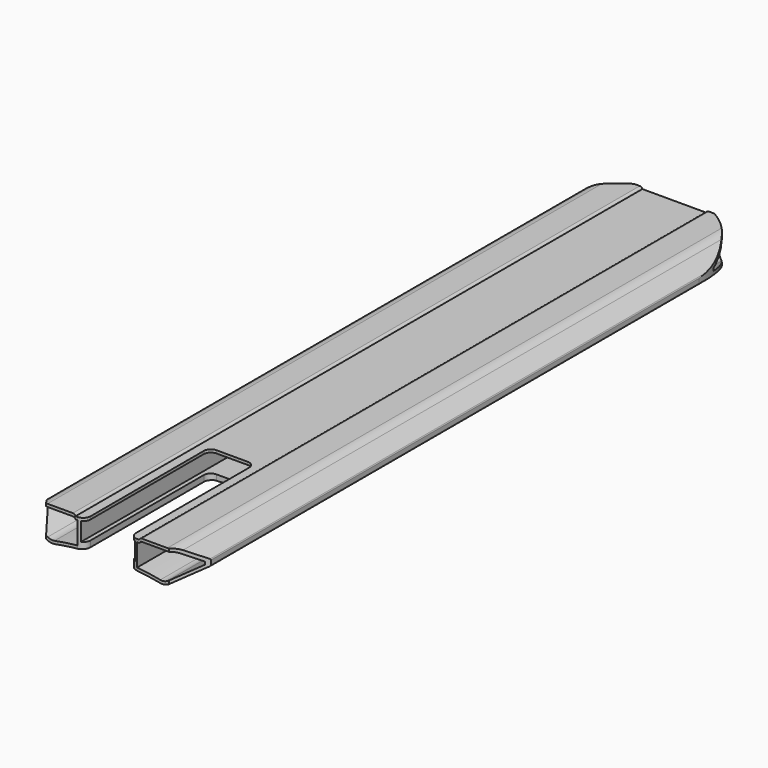
from build123d import *

# Parameters (mm, degrees)
F2_DEPTH       = 250
F3_W           = 38
F3_H           = 13
F4_DEPTH       = 250
F5_R           = 9
F6_R           = 1
F7_T1_DEPTH    = 509.3674969976
F9_DEPTH       = 500.001
F12_DEPTH      = 13.5192964571
F12_DEPTH_BACK = 10.001
F13_T1_DEPTH   = 2
F13_T6_DEPTH   = 16.7634354909
F13_S7_R       = 200
F13_T8_DEPTH   = 11
F13_T12_DEPTH  = 16.7632527384
F13_S13_R      = 200
F13_T14_DEPTH  = 11
F13_T15_DEPTH  = 29.2634354909
F13_T17_DEPTH  = 27
F13_T19_DEPTH  = 29.2632527384
F14_DEPTH      = 13.5192964571
F14_DEPTH_BACK = 10.001


# Not quite as in the source:
# - a fillet or chamfer that OpenCascade refuses, or shapes differently, is made with other operations: its cross-section is extruded or revolved along the edge and cut away or added


with BuildPart() as f2:
    # F0 (on Front) → F2 (new body, symmetric)
    with BuildSketch(Plane.XZ):
        with BuildLine():
            Line((-22.5004640741, 10), (-45.5824640741, 10))
            Line((-45.5824640741, 10), (-57.5, 0))
            Line((-57.5, 0), (-57.5, -4))
            Line((-57.5, -4), (-40.1794919243, -14))
            ThreePointArc((-40.1794919243, -14), (0.0006744682, -9.9223168214), (40.1808408606, -14))
            Line((40.1808408606, -14), (57.5, -4.0007788087))
            Line((57.5, -4.0007788087), (57.5, -0.0007788087))
            Line((57.5, -0.0007788087), (45.5815359259, 10))
            Line((45.5815359259, 10), (22.4995359259, 10))
            Line((22.4995359259, 10), (22.4995359259, 8.7))
            Line((22.4995359259, 8.7), (-22.5004640741, 8.7))
            Line((-22.5004640741, 8.7), (-22.5004640741, 10))
        make_face()
    extrude(amount=F2_DEPTH, both=True)

    # F3 (on Front) → F4 (cut, symmetric)
    with BuildSketch(Plane.XZ):
        with Locations((0, 0.2)):
            Rectangle(F3_W, F3_H)
    extrude(amount=F4_DEPTH, both=True, mode=Mode.SUBTRACT)

    # F5
    f5_edges = [f2.edges().sort_by_distance(p)[0] for p in [
        (45.581536, 0, 10),
        (40.180841, 0, -14),
        (-45.582464, 0, 10),
        (-40.179492, 0, -14),
    ]]
    fillet(f5_edges, radius=F5_R)

    # F6
    f6_edges = [f2.edges().sort_by_distance(p)[0] for p in [
        (57.5, 0, -0.000779),
        (57.5, 0, -4.000779),
        (-57.5, 0, 0),
        (-57.5, 0, -4),
    ]]
    fillet(f6_edges, radius=F6_R)

    # F7: fillet of radius 2 on 2 edges, made by hand

    # F7_s2 → F7_t1 (cut)
    with BuildSketch(Plane.XZ.offset(-254.6837484988)):
        with BuildLine():
            ThreePointArc((24.3730353255, 10), (23.2328599004, 9.6431676725), (22.4995359259, 8.7))
            Line((22.4995359259, 8.7), (22.4995359259, 10))
            Line((22.4995359259, 10), (24.3730353255, 10))
        make_face()
        with BuildLine():
            ThreePointArc((-22.5004640741, 8.7), (-23.2337880485, 9.6431676725), (-24.3739634736, 10))
            Line((-24.3739634736, 10), (-22.5004640741, 10))
            Line((-22.5004640741, 10), (-22.5004640741, 8.7))
        make_face()
    extrude(amount=F7_T1_DEPTH, mode=Mode.SUBTRACT)

    # F8 (on face) → F9 (cut, through all)
    with BuildSketch(Plane.XZ.offset(250)):
        with BuildLine():
            Line((-21, -9.0169369236), (-21, 6.6999997944))
            Line((-21, 6.6999997944), (-22.5004640741, 6.6999997944))
            ThreePointArc((-22.5004640741, 6.6999997944), (-23.2337879899, 7.6431676078), (-24.3739634736, 8))
            Line((-24.3739634736, 8), (-42.3067319657, 8))
            ThreePointArc((-42.3067319657, 8), (-44.7008729689, 7.5778483455), (-46.8062452335, 6.3623111018))
            Line((-46.8062452335, 6.3623111018), (-55.5, -0.9326153163))
            Line((-55.5, -0.9326153163), (-55.5, -2.8452994616))
            Line((-55.5, -2.8452994616), (-42.102284203, -10.5804742836))
            ThreePointArc((-42.102284203, -10.5804742836), (-39.7790708711, -11.4186713119), (-37.3093621422, -11.3978569477))
            ThreePointArc((-37.3093621422, -11.3978569477), (-29.178975147, -10.0409819041), (-21, -9.0169369236))
        make_face()
        with BuildLine():
            Line((22.5004640741, 6.6999997944), (21, 6.6999997944))
            Line((21, 6.6999997944), (21, -9.0169369236))
            ThreePointArc((21, -9.0169369236), (29.178975147, -10.0409819041), (37.3093621422, -11.3978569477))
            ThreePointArc((37.3093621422, -11.3978569477), (39.7790708711, -11.4186713119), (42.102284203, -10.5804742836))
            Line((42.102284203, -10.5804742836), (55.5, -2.8452994616))
            Line((55.5, -2.8452994616), (55.5, -0.9326153163))
            Line((55.5, -0.9326153163), (46.8062452335, 6.3623111018))
            ThreePointArc((46.8062452335, 6.3623111018), (44.7008729689, 7.5778483455), (42.3067319657, 8))
            Line((42.3067319657, 8), (24.3739634736, 8))
            ThreePointArc((24.3739634736, 8), (23.2337879899, 7.6431676078), (22.5004640741, 6.6999997944))
        make_face()
    extrude(amount=-F9_DEPTH, mode=Mode.SUBTRACT)

    # F11 (on Top) → F12 (cut, two sides)
    with BuildSketch(Plane.XY) as f12_sk:
        Polygon((-68.0004640741, -346), (67.9995359259, -346), (67.9995359259, -216), (43.2970899738, -250), (15.9995359259, -250), (15.9995359259, -140), (-16.0004640741, -140), (-16.0004640741, -250), (-43.2980181219, -250), (-68.0004640741, -216), align=None)
    extrude(amount=-F12_DEPTH, mode=Mode.SUBTRACT)
    extrude(f12_sk.sketch, amount=F12_DEPTH_BACK, mode=Mode.SUBTRACT)

    # F13: fillet of radius 5 on 8 edges, made by hand

    # F13_s2 → F13_t1 (join)
    with BuildSketch(Plane.XY.offset(6.7)):
        with BuildLine():
            ThreePointArc((-11.0004640741, -140), (-14.53599798, -141.4644660941), (-16.0004640741, -145))
            Line((-16.0004640741, -145), (-16.0004640741, -140))
            Line((-16.0004640741, -140), (-11.0004640741, -140))
        make_face()
        with BuildLine():
            ThreePointArc((15.9995359259, -145), (14.5350698319, -141.4644660941), (10.9995359259, -140))
            Line((10.9995359259, -140), (15.9995359259, -140))
            Line((15.9995359259, -140), (15.9995359259, -145))
        make_face()
    extrude(amount=F13_T1_DEPTH)


with BuildPart() as f13_tool4:
    # F13_s5 → F13_t6 (new body)
    with BuildSketch(Plane.XY.offset(-23.0634354909)):
        with BuildLine():
            ThreePointArc((-16.0004640741, -145), (-14.53599798, -141.4644660941), (-11.0004640741, -140))
            Line((-11.0004640741, -140), (-16.0004640741, -140))
            Line((-16.0004640741, -140), (-16.0004640741, -145))
        make_face()
    extrude(amount=F13_T6_DEPTH)

    # F13_s7 → F13_t8 (cut, symmetric)
    with BuildSketch(Plane.XZ.offset(142.5)):
        with Locations((0.0006744682, -209.9223168214)):
            Circle(F13_S7_R)
    extrude(amount=F13_T8_DEPTH, both=True, mode=Mode.SUBTRACT)


with BuildPart() as f2_1:
    add(f2.part)

    # F13_t3: union F13_tool4
    add(f13_tool4.part)


with BuildPart() as f13_tool10:
    # F13_s11 → F13_t12 (new body)
    with BuildSketch(Plane.XY.offset(-23.0632527384)):
        with BuildLine():
            ThreePointArc((15.9995359259, -145), (14.5350698319, -141.4644660941), (10.9995359259, -140))
            Line((10.9995359259, -140), (15.9995359259, -140))
            Line((15.9995359259, -140), (15.9995359259, -145))
        make_face()
    extrude(amount=F13_T12_DEPTH)

    # F13_s13 → F13_t14 (cut, symmetric)
    with BuildSketch(Plane.XZ.offset(142.5)):
        with Locations((0.0006744682, -209.9223168214)):
            Circle(F13_S13_R)
    extrude(amount=F13_T14_DEPTH, both=True, mode=Mode.SUBTRACT)


with BuildPart() as f2_2:
    add(f2_1.part)

    # F13_t9: union F13_tool10
    add(f13_tool10.part)

    # F13_s16 → F13_t15 (cut)
    with BuildSketch(Plane.XY.offset(-23.0634354909)):
        with BuildLine():
            ThreePointArc((-21.0004640741, -250), (-17.4649301681, -248.5355339059), (-16.0004640741, -245))
            Line((-16.0004640741, -245), (-16.0004640741, -250))
            Line((-16.0004640741, -250), (-21.0004640741, -250))
        make_face()
    extrude(amount=F13_T15_DEPTH, mode=Mode.SUBTRACT)

    # F13_s18 → F13_t17 (cut)
    with BuildSketch(Plane.XY.offset(-5.8)):
        with BuildLine():
            ThreePointArc((20.9995359259, -250), (17.46400202, -248.5355339059), (15.9995359259, -245))
            Line((15.9995359259, -245), (15.9995359259, -250))
            Line((15.9995359259, -250), (20.9995359259, -250))
        make_face()
        with BuildLine():
            ThreePointArc((-16.0004640741, -245), (-17.4649301681, -248.5355339059), (-21.0004640741, -250))
            Line((-21.0004640741, -250), (-16.0004640741, -250))
            Line((-16.0004640741, -250), (-16.0004640741, -245))
        make_face()
    extrude(amount=F13_T17_DEPTH, mode=Mode.SUBTRACT)

    # F13_s20 → F13_t19 (cut)
    with BuildSketch(Plane.XY.offset(-23.0632527384)):
        with BuildLine():
            ThreePointArc((20.9995359259, -250), (17.46400202, -248.5355339059), (15.9995359259, -245))
            Line((15.9995359259, -245), (15.9995359259, -250))
            Line((15.9995359259, -250), (20.9995359259, -250))
        make_face()
    extrude(amount=F13_T19_DEPTH, mode=Mode.SUBTRACT)

    # F10 (on Top) → F14 (cut, two sides)
    with BuildSketch(Plane.XY) as f14_sk:
        with BuildLine():
            ThreePointArc((-57.5, 200), (0, 257.5), (57.5, 200))
            Line((57.5, 200), (57.5, 280))
            Line((57.5, 280), (-57.5, 280))
            Line((-57.5, 280), (-57.5, 200))
        make_face()
    extrude(amount=-F14_DEPTH, mode=Mode.SUBTRACT)
    extrude(f14_sk.sketch, amount=F14_DEPTH_BACK, mode=Mode.SUBTRACT)


solid = f2_2.part
